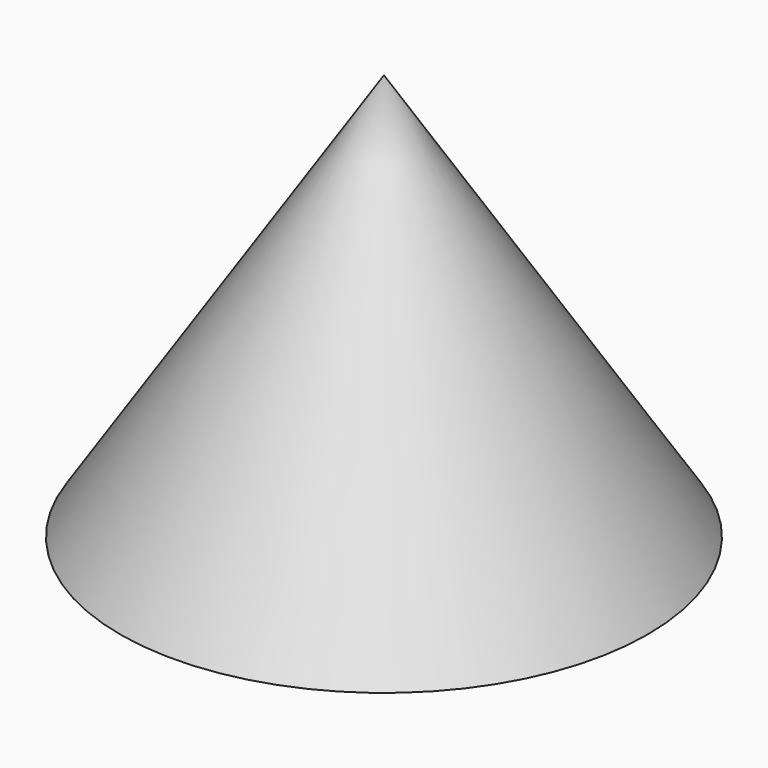
from build123d import *


# Not quite as in the source:
# - the program builds the solid bodies; features that only make, move or delete a surface that nothing else refers to are left out


with BuildPart() as f1:
    # F0 (on Front) → F1 (revolve)
    with BuildSketch(Plane.XZ):
        Polygon((-10.7847582549, -10.6004029512), (-31.6168554127, 21.4773397893), (-31.6168554127, -10.6004029512), align=None)
    revolve(axis=Axis((-31.6168554127, 0, 5.438468419), (0, 0, -1)))


solid = f1.part
